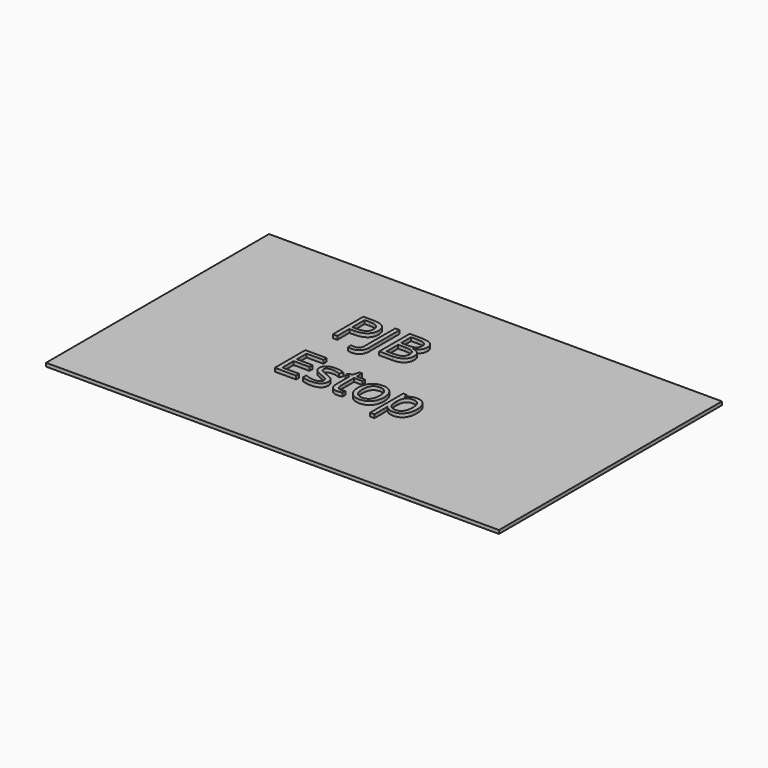
from build123d import *

# Parameters (mm, degrees)
F0_W         = 165.1
F0_H         = 101.6
F1_DEPTH     = 1.27
F2_TEXT_SIZE = 19.4473023089
F3_DEPTH     = 1.27


# Not quite as in the source:
# - Text() gives the source's letters only with a copy of the font that has no kerning and outlines rounded to 1/6400 em; it was checked with that copy


with BuildPart() as f1:
    # F0 (on Top) → F1 (new body)
    with BuildSketch(Plane.XY):
        with Locations((10.7107372791, -6.4242898051)):
            Rectangle(F0_W, F0_H)
    extrude(amount=F1_DEPTH)

    # F2 (on face) → F3 (join)
    with BuildSketch(Plane.XY.offset(1.27)):
        with Locations((-19.4334653116, 5.5788506149)):
            Text('PJB', F2_TEXT_SIZE, font='Open Sans', text_align=(TextAlign.LEFT, TextAlign.BOTTOM))
        with Locations((-19.4334653116, -20.8694805252)):
            Text('Estop', F2_TEXT_SIZE, font='Open Sans', text_align=(TextAlign.LEFT, TextAlign.BOTTOM))
    extrude(amount=F3_DEPTH)


solid = f1.part
